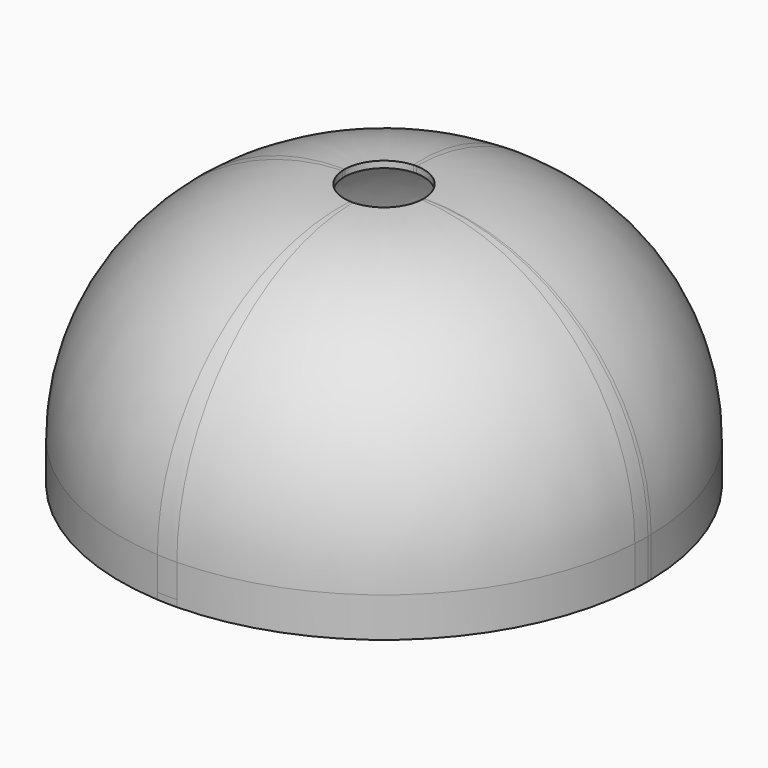
from build123d import *

# Parameters (mm, degrees)
F1_DEPTH = 40
F2_R     = 34
F3_T     = -1
F4_DEPTH = 1


# Not quite as in the source:
# - a shell that OpenCascade refuses in one call is made with other operations: the cavity is built on its own and cut out
# - a feature names something its author has since deleted; it is built from what else it names


with BuildPart() as f1:
    # F0 (on Top) → F1 (new body)
    with BuildSketch(Plane.XY):
        with BuildLine():
            Line((37, 0.6), (39.9954997468, 0.6))
            ThreePointArc((39.9954997468, 0.6), (28.2842712475, 28.2842712475), (0.6, 39.9954997468))
            Line((0.6, 39.9954997468), (0.6, 37))
            Line((0.6, 37), (-2.4, 37))
            Line((-2.4, 37), (-2.4, 39.9279350831))
            ThreePointArc((-2.4, 39.9279350831), (-28.9139450641, 27.6402565261), (-39.9954997468, 0.6))
            Line((-39.9954997468, 0.6), (-37, 0.6))
            Line((-37, 0.6), (-37, -2.4))
            Line((-37, -2.4), (-39.9279350831, -2.4))
            ThreePointArc((-39.9279350831, -2.4), (-28.2842712475, -28.2842712475), (-2.4, -39.9279350831))
            Line((-2.4, -39.9279350831), (-2.4, -37))
            Line((-2.4, -37), (0.6, -37))
            Line((0.6, -37), (0.6, -39.9954997468))
            ThreePointArc((0.6, -39.9954997468), (27.6402565261, -28.9139450641), (39.9279350831, -2.4))
            Line((39.9279350831, -2.4), (37, -2.4))
            Line((37, -2.4), (37, 0.6))
        make_face()
        with BuildLine():
            ThreePointArc((39.9279350831, -2.4), (39.9819797116, -1.2005408523), (40, 0))
            ThreePointArc((40, 0), (39.9988749209, 0.3000084383), (39.9954997468, 0.6))
            Line((39.9954997468, 0.6), (37, 0.6))
            Line((37, 0.6), (37, -2.4))
            Line((37, -2.4), (39.9279350831, -2.4))
        make_face()
        with BuildLine():
            Line((37, 0.6), (39.9954997468, 0.6))
            ThreePointArc((39.9954997468, 0.6), (28.2842712475, 28.2842712475), (0.6, 39.9954997468))
            Line((0.6, 39.9954997468), (0.6, 37))
            Line((0.6, 37), (-2.4, 37))
            Line((-2.4, 37), (-2.4, 39.9279350831))
            ThreePointArc((-2.4, 39.9279350831), (-28.9139450641, 27.6402565261), (-39.9954997468, 0.6))
            Line((-39.9954997468, 0.6), (-37, 0.6))
            Line((-37, 0.6), (-37, -2.4))
            Line((-37, -2.4), (-39.9279350831, -2.4))
            ThreePointArc((-39.9279350831, -2.4), (-28.2842712475, -28.2842712475), (-2.4, -39.9279350831))
            Line((-2.4, -39.9279350831), (-2.4, -37))
            Line((-2.4, -37), (0.6, -37))
            Line((0.6, -37), (0.6, -39.9954997468))
            ThreePointArc((0.6, -39.9954997468), (27.6402565261, -28.9139450641), (39.9279350831, -2.4))
            Line((39.9279350831, -2.4), (37, -2.4))
            Line((37, -2.4), (37, 0.6))
        make_face()
        with BuildLine():
            Line((37, 0.6), (39.9954997468, 0.6))
            ThreePointArc((39.9954997468, 0.6), (28.2842712475, 28.2842712475), (0.6, 39.9954997468))
            Line((0.6, 39.9954997468), (0.6, 37))
            Line((0.6, 37), (-2.4, 37))
            Line((-2.4, 37), (-2.4, 39.9279350831))
            ThreePointArc((-2.4, 39.9279350831), (-28.9139450641, 27.6402565261), (-39.9954997468, 0.6))
            Line((-39.9954997468, 0.6), (-37, 0.6))
            Line((-37, 0.6), (-37, -2.4))
            Line((-37, -2.4), (-39.9279350831, -2.4))
            ThreePointArc((-39.9279350831, -2.4), (-28.2842712475, -28.2842712475), (-2.4, -39.9279350831))
            Line((-2.4, -39.9279350831), (-2.4, -37))
            Line((-2.4, -37), (0.6, -37))
            Line((0.6, -37), (0.6, -39.9954997468))
            ThreePointArc((0.6, -39.9954997468), (27.6402565261, -28.9139450641), (39.9279350831, -2.4))
            Line((39.9279350831, -2.4), (37, -2.4))
            Line((37, -2.4), (37, 0.6))
        make_face()
        with BuildLine():
            Line((37, 0.6), (39.9954997468, 0.6))
            ThreePointArc((39.9954997468, 0.6), (28.2842712475, 28.2842712475), (0.6, 39.9954997468))
            Line((0.6, 39.9954997468), (0.6, 37))
            Line((0.6, 37), (-2.4, 37))
            Line((-2.4, 37), (-2.4, 39.9279350831))
            ThreePointArc((-2.4, 39.9279350831), (-28.9139450641, 27.6402565261), (-39.9954997468, 0.6))
            Line((-39.9954997468, 0.6), (-37, 0.6))
            Line((-37, 0.6), (-37, -2.4))
            Line((-37, -2.4), (-39.9279350831, -2.4))
            ThreePointArc((-39.9279350831, -2.4), (-28.2842712475, -28.2842712475), (-2.4, -39.9279350831))
            Line((-2.4, -39.9279350831), (-2.4, -37))
            Line((-2.4, -37), (0.6, -37))
            Line((0.6, -37), (0.6, -39.9954997468))
            ThreePointArc((0.6, -39.9954997468), (27.6402565261, -28.9139450641), (39.9279350831, -2.4))
            Line((39.9279350831, -2.4), (37, -2.4))
            Line((37, -2.4), (37, 0.6))
        make_face()
        with BuildLine():
            ThreePointArc((39.9279350831, -2.4), (39.9819797116, -1.2005408523), (40, 0))
            ThreePointArc((40, 0), (39.9988749209, 0.3000084383), (39.9954997468, 0.6))
            Line((39.9954997468, 0.6), (37, 0.6))
            Line((37, 0.6), (37, -2.4))
            Line((37, -2.4), (39.9279350831, -2.4))
        make_face()
        with BuildLine():
            ThreePointArc((-2.4, -39.9279350831), (-0.9006338024, -39.989859449), (0.6, -39.9954997468))
            Line((0.6, -39.9954997468), (0.6, -37))
            Line((0.6, -37), (-2.4, -37))
            Line((-2.4, -37), (-2.4, -39.9279350831))
        make_face()
        with BuildLine():
            Line((-37, 0.6), (-39.9954997468, 0.6))
            ThreePointArc((-39.9954997468, 0.6), (-39.989859449, -0.9006338024), (-39.9279350831, -2.4))
            Line((-39.9279350831, -2.4), (-37, -2.4))
            Line((-37, -2.4), (-37, 0.6))
        make_face()
        with BuildLine():
            Line((0.6, 37), (0.6, 39.9954997468))
            ThreePointArc((0.6, 39.9954997468), (-0.9006338024, 39.989859449), (-2.4, 39.9279350831))
            Line((-2.4, 39.9279350831), (-2.4, 37))
            Line((-2.4, 37), (0.6, 37))
        make_face()
        with BuildLine():
            Line((37, 0.6), (39.9954997468, 0.6))
            ThreePointArc((39.9954997468, 0.6), (28.2842712475, 28.2842712475), (0.6, 39.9954997468))
            Line((0.6, 39.9954997468), (0.6, 37))
            Line((0.6, 37), (-2.4, 37))
            Line((-2.4, 37), (-2.4, 39.9279350831))
            ThreePointArc((-2.4, 39.9279350831), (-28.9139450641, 27.6402565261), (-39.9954997468, 0.6))
            Line((-39.9954997468, 0.6), (-37, 0.6))
            Line((-37, 0.6), (-37, -2.4))
            Line((-37, -2.4), (-39.9279350831, -2.4))
            ThreePointArc((-39.9279350831, -2.4), (-28.2842712475, -28.2842712475), (-2.4, -39.9279350831))
            Line((-2.4, -39.9279350831), (-2.4, -37))
            Line((-2.4, -37), (0.6, -37))
            Line((0.6, -37), (0.6, -39.9954997468))
            ThreePointArc((0.6, -39.9954997468), (27.6402565261, -28.9139450641), (39.9279350831, -2.4))
            Line((39.9279350831, -2.4), (37, -2.4))
            Line((37, -2.4), (37, 0.6))
        make_face()
        with BuildLine():
            Line((37, 0.6), (39.9954997468, 0.6))
            ThreePointArc((39.9954997468, 0.6), (28.2842712475, 28.2842712475), (0.6, 39.9954997468))
            Line((0.6, 39.9954997468), (0.6, 37))
            Line((0.6, 37), (-2.4, 37))
            Line((-2.4, 37), (-2.4, 39.9279350831))
            ThreePointArc((-2.4, 39.9279350831), (-28.9139450641, 27.6402565261), (-39.9954997468, 0.6))
            Line((-39.9954997468, 0.6), (-37, 0.6))
            Line((-37, 0.6), (-37, -2.4))
            Line((-37, -2.4), (-39.9279350831, -2.4))
            ThreePointArc((-39.9279350831, -2.4), (-28.2842712475, -28.2842712475), (-2.4, -39.9279350831))
            Line((-2.4, -39.9279350831), (-2.4, -37))
            Line((-2.4, -37), (0.6, -37))
            Line((0.6, -37), (0.6, -39.9954997468))
            ThreePointArc((0.6, -39.9954997468), (27.6402565261, -28.9139450641), (39.9279350831, -2.4))
            Line((39.9279350831, -2.4), (37, -2.4))
            Line((37, -2.4), (37, 0.6))
        make_face()
    extrude(amount=F1_DEPTH)

    # F2
    f2_edges = [f1.edges().sort_by_distance(p)[0] for p in [
        (-0.6, -39.9955, 40),
    ]]
    fillet(f2_edges, radius=F2_R)

    # F3: a shell. OpenCascade refuses it in one call, so the cavity is built on its own and cut out:
    # the body offset inwards by the wall thickness, plus a prism from it out through each open face.
    f3_core = offset(f1.part, amount=F3_T, mode=Mode.PRIVATE)
    f3_exits = [f3_core.faces().sort_by_distance(p)[0] for p in [
        (0, 0, 39),
        (0, 0, 1),
    ]]
    add(f3_core, mode=Mode.SUBTRACT)
    extrude(f3_exits, amount=-F3_T, mode=Mode.SUBTRACT)

    # F0 (on Top) → F4 (join)
    with BuildSketch(Plane.XY):
        with BuildLine():
            ThreePointArc((39.9279350831, -2.4), (39.9819797116, -1.2005408523), (40, 0))
            ThreePointArc((40, 0), (39.9988749209, 0.3000084383), (39.9954997468, 0.6))
            Line((39.9954997468, 0.6), (37, 0.6))
            Line((37, 0.6), (37, -2.4))
            Line((37, -2.4), (39.9279350831, -2.4))
        make_face()
        with BuildLine():
            Line((0.6, 37), (0.6, 39.9954997468))
            ThreePointArc((0.6, 39.9954997468), (-0.9006338024, 39.989859449), (-2.4, 39.9279350831))
            Line((-2.4, 39.9279350831), (-2.4, 37))
            Line((-2.4, 37), (0.6, 37))
        make_face()
        with BuildLine():
            Line((-37, 0.6), (-39.9954997468, 0.6))
            ThreePointArc((-39.9954997468, 0.6), (-39.989859449, -0.9006338024), (-39.9279350831, -2.4))
            Line((-39.9279350831, -2.4), (-37, -2.4))
            Line((-37, -2.4), (-37, 0.6))
        make_face()
        with BuildLine():
            ThreePointArc((-2.4, -39.9279350831), (-0.9006338024, -39.989859449), (0.6, -39.9954997468))
            Line((0.6, -39.9954997468), (0.6, -37))
            Line((0.6, -37), (-2.4, -37))
            Line((-2.4, -37), (-2.4, -39.9279350831))
        make_face()
    extrude(amount=F4_DEPTH)


solid = f1.part
